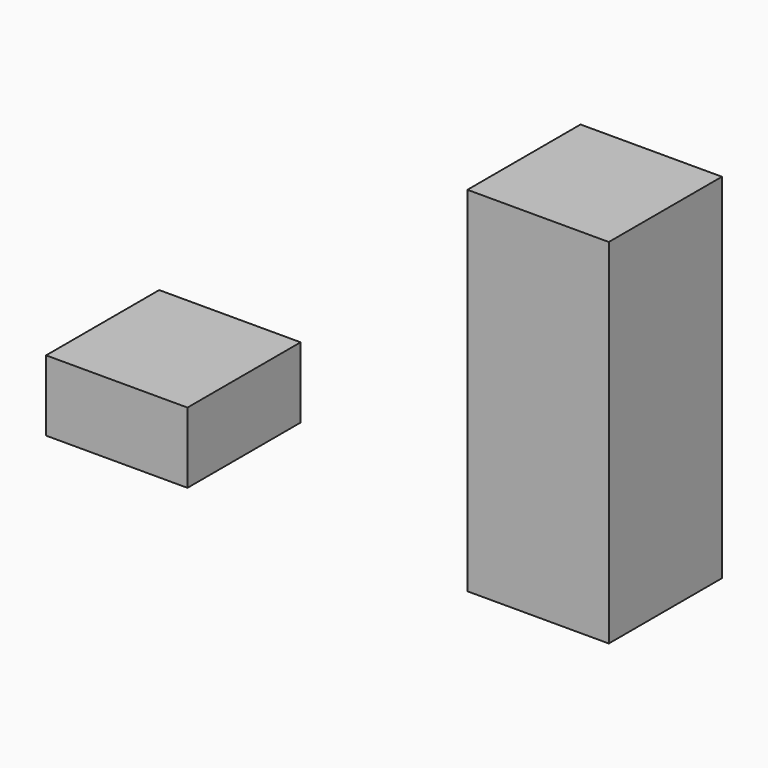
from build123d import *

# Parameters (mm, degrees)
F1_DEPTH = 6.35
F0_W     = 12.7
F0_H     = 12.7
F2_DEPTH = 31.75


# Not quite as in the source:
# - ends of sketch curves that miss each other by under 0.0002 mm in the source are joined


with BuildPart() as f1:
    # F0 (on Top) → F1 (new body)
    with BuildSketch(Plane.XY):
        Polygon((-14.0986793399, 6.1743884951), (-26.7986793399, 6.1743884951), (-26.7986777842, -6.5256115049), (-14.0986793399, -6.5256115049), align=None)
    extrude(amount=F1_DEPTH)


with BuildPart() as f2:
    # F0 (on Top) → F2 (new body)
    with BuildSketch(Plane.XY):
        with Locations((17.397325097, -0.1756115049)):
            Rectangle(F0_W, F0_H)
    extrude(amount=F2_DEPTH)


solid = Compound([f1.part, f2.part])
